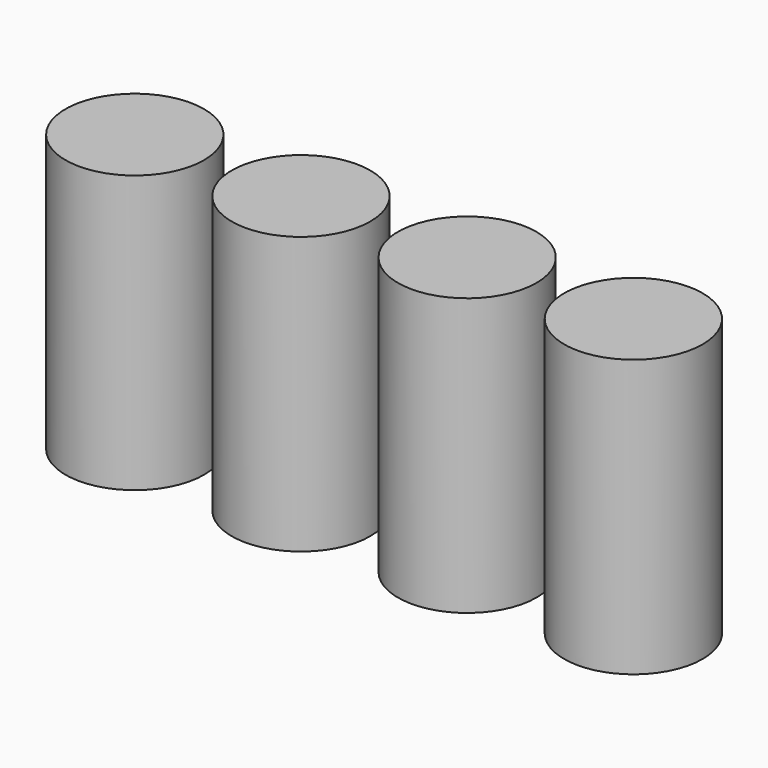
from build123d import *

# Parameters (mm, degrees)
F0_R     = 5
F1_DEPTH = 20


# Not quite as in the source:
# - the program builds the solid bodies; features that only make, move or delete a surface that nothing else refers to are left out


with BuildPart() as f1:
    # F0 (on Top) → F1 (new body)
    with BuildSketch(Plane.XY):
        with Locations((-150, -11)):
            Circle(F0_R)
    extrude(amount=F1_DEPTH)


with BuildPart() as f1b:
    # F0 (on Top) → F1, piece 2 (new body)
    with BuildSketch(Plane.XY):
        with Locations((-138, -11)):
            Circle(F0_R)
    extrude(amount=F1_DEPTH)


with BuildPart() as f1c:
    # F0 (on Top) → F1, piece 3 (new body)
    with BuildSketch(Plane.XY):
        with Locations((-126, -11)):
            Circle(F0_R)
    extrude(amount=F1_DEPTH)


with BuildPart() as f1d:
    # F0 (on Top) → F1, piece 4 (new body)
    with BuildSketch(Plane.XY):
        with Locations((-114, -11)):
            Circle(F0_R)
    extrude(amount=F1_DEPTH)


solid = Compound([f1.part, f1b.part, f1c.part, f1d.part])
